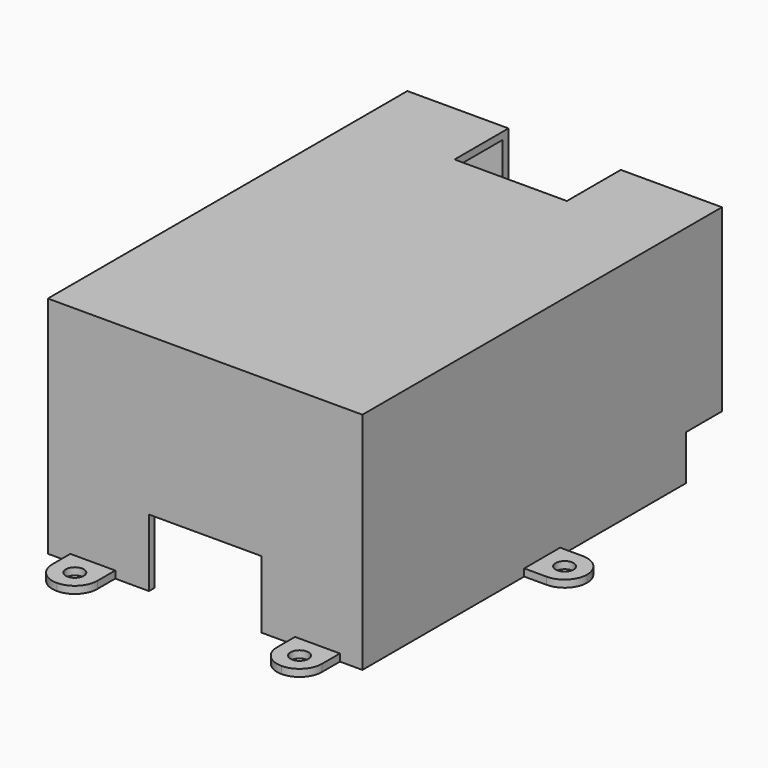
from build123d import *

# Parameters (mm, degrees)
F0_W      = 70
F0_H      = 100
F1_DEPTH  = 50
F2_T      = -1.6
F3_W      = 10
F3_H      = 10
F4_DEPTH  = 70.001
F5_W      = 10
F5_H      = 10
F5_R      = 2
F6_DEPTH  = 1.6
F7_R      = 4.99999
F8_W      = 25
F8_H      = 15
F9_DEPTH  = 50.001
F10_W     = 25
F10_H     = 15
F11_DEPTH = 100.001


# Not quite as in the source:
# - a fillet or chamfer is up to 0.001 mm smaller than in the source, because OpenCascade refuses the exact size


with BuildPart() as f1:
    # F0 (on Top) → F1 (new body)
    with BuildSketch(Plane.XY):
        Rectangle(F0_W, F0_H)
    extrude(amount=F1_DEPTH)

    # F2
    f2_openings = [f1.faces().sort_by_distance(p)[0] for p in [
        (0, 0, 0),
    ]]
    offset(amount=F2_T, openings=f2_openings)

    # F3 (on face) → F4 (cut, through all)
    with BuildSketch(Plane.YZ.offset(35)):
        with Locations((45, 5)):
            Rectangle(F3_W, F3_H)
    extrude(amount=-F4_DEPTH, mode=Mode.SUBTRACT)

    # F5 (on Top) → F6 (join)
    with BuildSketch(Plane.XY):
        with Locations((40, 0)):
            Rectangle(F5_W, F5_H)
        with Locations((40, 0)):
            Circle(F5_R, mode=Mode.SUBTRACT)
        with Locations((-40, 0)):
            Rectangle(F5_W, F5_H)
        with Locations((-40, 0)):
            Circle(F5_R, mode=Mode.SUBTRACT)
        with Locations((-25, -55)):
            Rectangle(F5_W, F5_H)
        with Locations((-25, -55)):
            Circle(F5_R, mode=Mode.SUBTRACT)
        with Locations((25, -55)):
            Rectangle(F5_W, F5_H)
        with Locations((25, -55)):
            Circle(F5_R, mode=Mode.SUBTRACT)
    extrude(amount=F6_DEPTH)

    # F7 (radius 5 in the source; OpenCascade refuses exactly that, so slightly less here)
    f7_edges = [f1.edges().sort_by_distance(p)[0] for p in [
        (-45, -5, 0.8),
        (-45, 5, 0.8),
        (45, -5, 0.8),
        (45, 5, 0.8),
        (-30, -60, 0.8),
        (-20, -60, 0.8),
        (20, -60, 0.8),
        (30, -60, 0.8),
    ]]
    fillet(f7_edges, radius=F7_R)

    # F8 (on face) → F9 (cut, through all)
    with BuildSketch(Plane.XY.offset(50)):
        with Locations((0, 42.5)):
            Rectangle(F8_W, F8_H)
    extrude(amount=-F9_DEPTH, mode=Mode.SUBTRACT)

    # F10 (on face) → F11 (cut, through all)
    with BuildSketch(Plane.XZ.offset(50)):
        with Locations((0, 7.5)):
            Rectangle(F10_W, F10_H)
    extrude(amount=-F11_DEPTH, mode=Mode.SUBTRACT)


solid = f1.part
